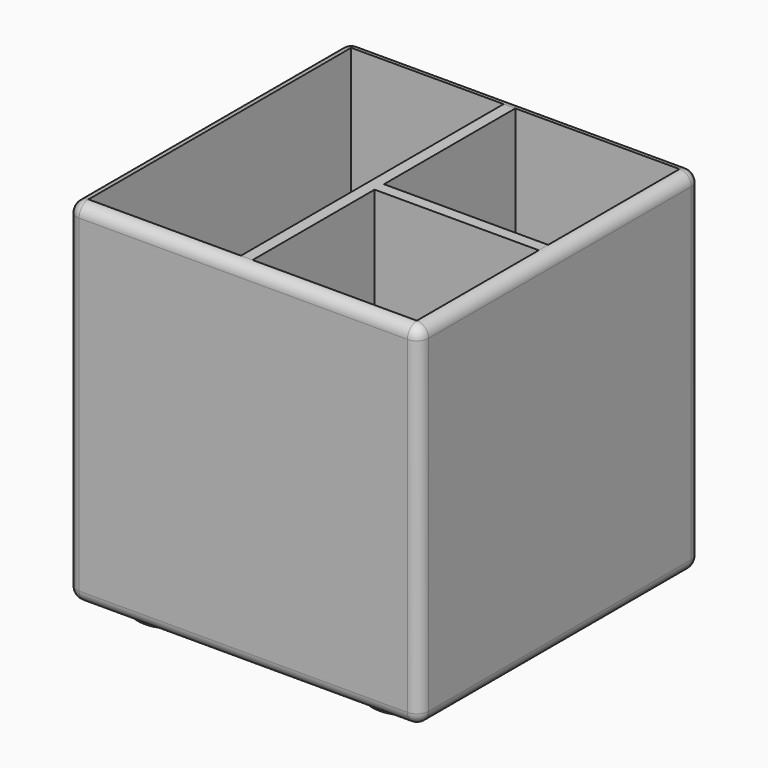
from build123d import *

# Parameters (mm, degrees)
F0_W      = 150
F0_H      = 150
F1_DEPTH  = 75
F2_W      = 140
F2_H      = 140
F3_DEPTH  = 140
F4_R      = 4.99999
F5_W      = 70
F5_H      = 140
F6_DEPTH  = 140
F7_W      = 65
F7_H      = 140
F8_DEPTH  = 140
F9_W      = 70
F9_H      = 70
F10_DEPTH = 140
F11_W     = 70
F11_H     = 65
F12_DEPTH = 140
F13_R     = 15
F14_DEPTH = 5


# Not quite as in the source:
# - a fillet or chamfer is up to 0.001 mm smaller than in the source, because OpenCascade refuses the exact size


with BuildPart() as f1:
    # F0 (on Front) → F1 (new body, symmetric)
    with BuildSketch(Plane.XZ):
        Rectangle(F0_W, F0_H)
    extrude(amount=F1_DEPTH, both=True)

    # F2 (on face) → F3 (cut)
    with BuildSketch(Plane.XY.offset(75)):
        Rectangle(F2_W, F2_H)
    extrude(amount=-F3_DEPTH, mode=Mode.SUBTRACT)

    # F4 (radius 5 in the source; OpenCascade refuses exactly that, so slightly less here)
    f4_edges = [f1.edges().sort_by_distance(p)[0] for p in [
        (0, -75, -75),
        (75, -75, 0),
        (0, -75, 75),
        (-75, -75, 0),
        (75, 0, -75),
        (75, 75, 0),
        (75, 0, 75),
        (-75, 75, 0),
        (-75, 0, -75),
        (-75, 0, 75),
        (0, 75, -75),
        (0, 75, 75),
    ]]
    fillet(f4_edges, radius=F4_R)

    # F5 (on face) → F6 (join)
    with BuildSketch(Plane.XY.offset(-65)):
        with Locations((-35, 0)):
            Rectangle(F5_W, F5_H)
    extrude(amount=F6_DEPTH)

    # F7 (on face) → F8 (cut)
    with BuildSketch(Plane.XY.offset(75)):
        with Locations((-37.5, 0)):
            Rectangle(F7_W, F7_H)
    extrude(amount=-F8_DEPTH, mode=Mode.SUBTRACT)

    # F9 (on face) → F10 (join)
    with BuildSketch(Plane.XY.offset(-65)):
        with Locations((35, -35)):
            Rectangle(F9_W, F9_H)
    extrude(amount=F10_DEPTH)

    # F11 (on face) → F12 (cut)
    with BuildSketch(Plane.XY.offset(75)):
        with Locations((35, -37.5)):
            Rectangle(F11_W, F11_H)
    extrude(amount=-F12_DEPTH, mode=Mode.SUBTRACT)

    # F13 (on face) → F14 (join)
    with BuildSketch(Plane(origin=(0, 0, -75), x_dir=(1, 0, 0), z_dir=(0, 0, -1))):
        with Locations((-50, 50)):
            Circle(F13_R)
        with Locations((50, 50)):
            Circle(F13_R)
        with Locations((50, -50)):
            Circle(F13_R)
        with Locations((-50, -50)):
            Circle(F13_R)
    extrude(amount=F14_DEPTH)


solid = f1.part
